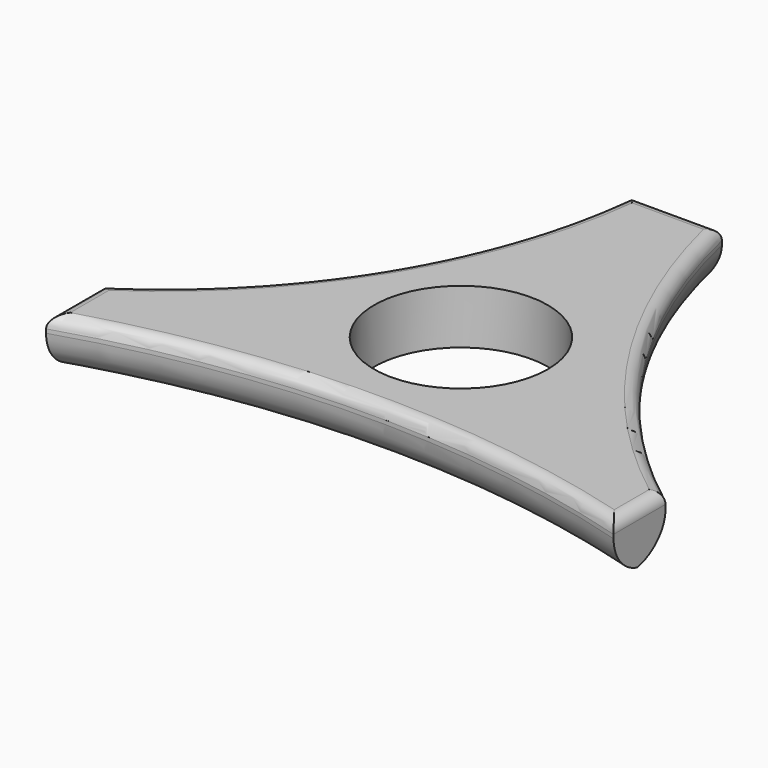
from build123d import *

# Parameters (mm, degrees)
F0_R        = 11.2
F1_DEPTH    = 7
F2_R        = 1.5
F3_T1_DEPTH = 36.7018774228
F3_T4_ANGLE = 72.934456587
F3_T6_ANGLE = 45.7548994245
F3_T8_ANGLE = 56.9956661229


# Not quite as in the source:
# - a fillet or chamfer that OpenCascade refuses, or shapes differently, is made with other operations: its cross-section is extruded or revolved along the edge and cut away or added


with BuildPart() as f1:
    # F0 (on Top) → F1 (new body)
    with BuildSketch(Plane.XY):
        with BuildLine():
            ThreePointArc((-6.1555781478, 35.1188629866), (-15.3560457965, 7.5552379901), (-35.5490386319, -13.3408159018))
            Line((-35.5490386319, -13.3408159018), (-35.5490386319, -22.4113118275))
            ThreePointArc((-35.5490386319, -22.4113118275), (0.6952562714, -16.6112557297), (37.0443966853, -21.713172521))
            Line((37.0443966853, -21.713172521), (37.0443966853, -13.3408159018))
            ThreePointArc((37.0443966853, -13.3408159018), (17.019752647, 8.1099477957), (5.546299275, 35.1188629866))
            Line((5.546299275, 35.1188629866), (-6.1555781478, 35.1188629866))
        make_face()
        Circle(F0_R, mode=Mode.SUBTRACT)
    extrude(amount=F1_DEPTH)

    # F2
    f2_edges = [f1.edges().sort_by_distance(p)[0] for p in [
        (-35.549039, -17.876064, 7),
        (0.695256, -16.611256, 7),
        (-15.356046, 7.555238, 7),
        (17.019753, 8.109948, 7),
        (37.044397, -17.526994, 7),
        (-0.304639, 35.118863, 7),
    ]]
    fillet(f2_edges, radius=F2_R)

    # F3: fillet of radius 5 on 6 edges, made by hand

    # F3_s2 → F3_t1 (cut)
    with BuildSketch(Plane.YZ.offset(-18.6555781478)):
        with BuildLine():
            ThreePointArc((30.1188629866, 0), (33.6543968925, 1.4644660941), (35.1188629866, 5))
            Line((35.1188629866, 5), (35.1188629866, 0))
            Line((35.1188629866, 0), (30.1188629866, 0))
        make_face()
    extrude(amount=F3_T1_DEPTH, mode=Mode.SUBTRACT)

    # F3_s3 → F3_t4 (revolve, cut)
    with BuildSketch(Plane(origin=(-4.3701670653, 47.7604075053, 0), x_dir=(0, 0, 1), z_dir=(-0.0911212144, 0.9958398085, 0))):
        with BuildLine():
            ThreePointArc((0, 3.2563304614), (1.4644660941, -0.2792034445), (5, -1.7436695386))
            Line((5, -1.7436695386), (0, -1.7436695386))
            Line((0, -1.7436695386), (0, 3.2563304614))
        make_face()
    revolve(axis=Axis((-71.5118436224, 41.6168178894, 0), (0, 0, -1)), revolution_arc=F3_T4_ANGLE, mode=Mode.SUBTRACT)

    # F3_s5 → F3_t6 (revolve, cut)
    with BuildSketch(Plane(origin=(-49.5559041376, -21.4739784979, 0), x_dir=(0, 0, 1), z_dir=(-0.9175572913, -0.3976035931, 0))):
        with BuildLine():
            ThreePointArc((0, -0.7975032251), (1.4644660941, -4.333037131), (5, -5.7975032251))
            Line((5, -5.7975032251), (0, -5.7975032251))
            Line((0, -5.7975032251), (0, -0.7975032251))
        make_face()
    revolve(axis=Axis((1.8836501986, -140.182005695, 0), (0, 0, -1)), revolution_arc=F3_T6_ANGLE, mode=Mode.SUBTRACT)

    # F3_s7 → F3_t8 (revolve, cut)
    with BuildSketch(Plane(origin=(45.161339961, -24.4990526211, 0), x_dir=(0, 0, 1), z_dir=(0.8789929725, -0.4768347243, 0))):
        with BuildLine():
            ThreePointArc((5, -5.0138287397), (1.4644660941, -3.5493626456), (0, -0.0138287397))
            Line((0, -0.0138287397), (0, -5.0138287397))
            Line((0, -5.0138287397), (5, -5.0138287397))
        make_face()
    revolve(axis=Axis((87.8129156777, 54.1244901178, 0), (0, 0, -1)), revolution_arc=F3_T8_ANGLE, mode=Mode.SUBTRACT)


solid = f1.part
